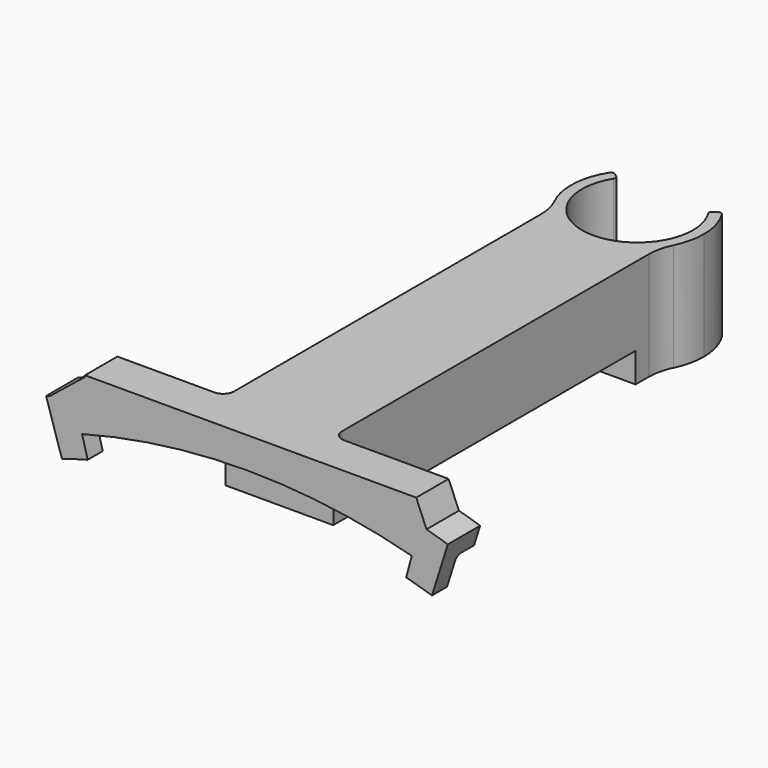
from build123d import *

# Parameters (mm, degrees)
F1_DEPTH       = 25.4
F2_DEPTH       = 25.4
F3_R           = 12.7
F4_R           = 0.762
F6_DEPTH       = 88.9
F7_W           = 25.4
F7_H           = 18.415
F8_DEPTH       = 2.54
F10_W          = 9.525
F10_H          = 3.81
F10_W_2        = 4.445
F10_H_2        = 5.08
F11_ANGLE_BACK = 17.5
F11_ANGLE      = 35
F12_R          = 1.27
F13_DEPTH      = 38.1
F14_R          = 2.54
F15_ANGLE_BACK = 15
F15_ANGLE      = 30
F16_T1_DEPTH   = 9.525
F16_T6_DEPTH   = 9.525


# Not quite as in the source:
# - a fillet or chamfer that OpenCascade refuses, or shapes differently, is made with other operations: its cross-section is extruded or revolved along the edge and cut away or added


with BuildPart() as f1:
    # F0 (on Top) → F1 (new body)
    with BuildSketch(Plane.XY):
        with BuildLine():
            ThreePointArc((12.7, -9.0953637091), (14.8728333044, -4.7764495705), (15.621, 0))
            ThreePointArc((15.621, 0), (14.8980124876, 4.6973252941), (12.7959740838, 8.9598375122))
            Line((12.7959740838, 8.9598375122), (10.7153278913, 7.5029533639))
            ThreePointArc((10.7153278913, 7.5029533639), (12.4755714327, 3.9335325633), (13.081, 0))
            ThreePointArc((13.081, 0), (-3.9335325633, -12.4755714327), (-10.7153278913, 7.5029533639))
            Line((-10.7153278913, 7.5029533639), (-12.7959740838, 8.9598375122))
            ThreePointArc((-12.7959740838, 8.9598375122), (-15.6207793149, -0.0830336901), (-12.7, -9.0953637091))
            ThreePointArc((-12.7, -9.0953637091), (0, -15.621), (12.7, -9.0953637091))
        make_face()
    extrude(amount=-F1_DEPTH)

    # F0 (on Top) → F2 (join, through all)
    with BuildSketch(Plane.XY):
        with BuildLine():
            Line((12.7, -16.4338), (12.7, -9.0953637091))
            ThreePointArc((12.7, -9.0953637091), (0, -15.621), (-12.7, -9.0953637091))
            Line((-12.7, -9.0953637091), (-12.7, -16.4338))
            Line((-12.7, -16.4338), (12.7, -16.4338))
        make_face()
    extrude(amount=-F2_DEPTH)

    # F3
    f3_edges = [f1.edges().sort_by_distance(p)[0] for p in [
        (-12.7, -9.095364, -12.7),
        (12.7, -9.095364, -12.7),
    ]]
    fillet(f3_edges, radius=F3_R)

    # F4
    f4_edges = [f1.edges().sort_by_distance(p)[0] for p in [
        (-12.795974, 8.959838, -12.7),
        (-10.715328, 7.502953, -12.7),
        (12.795974, 8.959838, -12.7),
        (10.715328, 7.502953, -12.7),
    ]]
    fillet(f4_edges, radius=F4_R)

    # F5 (on face) → F6 (join)
    with BuildSketch(Plane.XZ.offset(16.4338)):
        Polygon((10.16, -18.415), (12.7, -18.415), (12.7, 0), (-12.7, 0), (-12.7, -18.415), (-10.16, -18.415), (-10.16, -2.54), (10.16, -2.54), align=None)
    extrude(amount=F6_DEPTH)

    # F7 (on face) → F8 (join)
    with BuildSketch(Plane.XZ.offset(105.3338)):
        with Locations((0, -9.2075)):
            Rectangle(F7_W, F7_H)
    extrude(amount=-F8_DEPTH)

    # F10 (on Right) → F11 (revolve)
    with BuildSketch(Plane.YZ, mode=Mode.PRIVATE) as f11_sk:
        with Locations((-110.0963, -1.905)):
            Rectangle(F10_W, F10_H)
        Polygon((-105.3338, -3.81), (-114.8588, -3.81), (-114.8588, -7.3025), (-110.4138, -7.3025), (-110.4138, -4.7625), (-105.3338, -4.7625), align=None)
        with Locations((-112.6363, -9.8425)):
            Rectangle(F10_W_2, F10_H_2)
    revolve(f11_sk.sketch.rotate(Axis((0, -105.3338, -157.1625), (0, -1, 0)), -F11_ANGLE_BACK), axis=Axis((0, -105.3338, -157.1625), (0, -1, 0)), revolution_arc=F11_ANGLE)

    # F12
    f12_edges = [f1.edges().sort_by_distance(p)[0] for p in [
        (0, -110.4138, -4.7625),
    ]]
    fillet(f12_edges, radius=F12_R)

    # F10 (on Right) → F13 (join, symmetric)
    with BuildSketch(Plane.YZ):
        with Locations((-110.0963, -1.905)):
            Rectangle(F10_W, F10_H)
        Polygon((-105.3338, -3.81), (-114.8588, -3.81), (-114.8588, -7.3025), (-110.4138, -7.3025), (-110.4138, -4.7625), (-105.3338, -4.7625), align=None)
        with Locations((-112.6363, -9.8425)):
            Rectangle(F10_W_2, F10_H_2)
    extrude(amount=F13_DEPTH, both=True)

    # F14
    f14_edges = [f1.edges().sort_by_distance(p)[0] for p in [
        (-12.7, -105.3338, -2.646294),
        (12.7, -105.3338, -2.646294),
    ]]
    fillet(f14_edges, radius=F14_R)

    # F10 (on Right) → F15 (revolve, cut)
    with BuildSketch(Plane.YZ, mode=Mode.PRIVATE) as f15_sk:
        with Locations((-112.6363, -9.8425)):
            Rectangle(F10_W_2, F10_H_2)
    revolve(f15_sk.sketch.rotate(Axis((0, -114.8588, -157.1625), (0, 1, 0)), -F15_ANGLE_BACK), axis=Axis((0, -114.8588, -157.1625), (0, 1, 0)), revolution_arc=F15_ANGLE, mode=Mode.SUBTRACT)

    # F16: chamfer of 4.572 x 8.89 on 2 edges, made by hand

    # F16_s2 → F16_t1 (join)
    with BuildSketch(Plane.XZ.offset(105.3338)):
        with BuildLine():
            Line((-37.8226041978, -0.1454336847), (-46.6377637043, -7.2158622396))
            Line((-46.6377637043, -7.2158622396), (-46.5853156114, -7.3857505486))
            ThreePointArc((-46.5853156114, -7.3857505486), (-42.3555242037, -5.9996553472), (-38.0568969697, -4.8606003824))
            Line((-38.0568969697, -4.8606003824), (-37.9222, -4.6881040961))
            ThreePointArc((-37.9222, -4.6881040961), (-37.9222, -2.4167688904), (-37.6448041978, -0.1454336847))
            Line((-37.6448041978, -0.1454336847), (-37.8226041978, -0.1454336847))
        make_face()
    extrude(amount=F16_T1_DEPTH)


with BuildPart() as f16_tool4:
    # F16_s5 → F16_t6 (new body)
    with BuildSketch(Plane.XZ.offset(105.3338)):
        with BuildLine():
            Line((37.9624780483, 4.4650442814), (42.400178494, -6.1169884318))
            Line((42.400178494, -6.1169884318), (42.3523661957, -6.2882391956))
            ThreePointArc((42.3523661957, -6.2882391956), (40.2444090257, -5.4239631141), (38.0568969697, -4.8606003824))
            Line((38.0568969697, -4.8606003824), (37.9222, -4.6881040961))
            ThreePointArc((37.9222, -4.6881040961), (37.9222, -0.1115299073), (37.7846780483, 4.4650442814))
            Line((37.7846780483, 4.4650442814), (37.9624780483, 4.4650442814))
        make_face()
    extrude(amount=F16_T6_DEPTH)

    split(bisect_by=Plane.XY, keep=Keep.BOTTOM)


with BuildPart() as f1_1:
    add(f1.part)

    # F16_t3: union F16_tool4
    add(f16_tool4.part)


solid = f1_1.part
